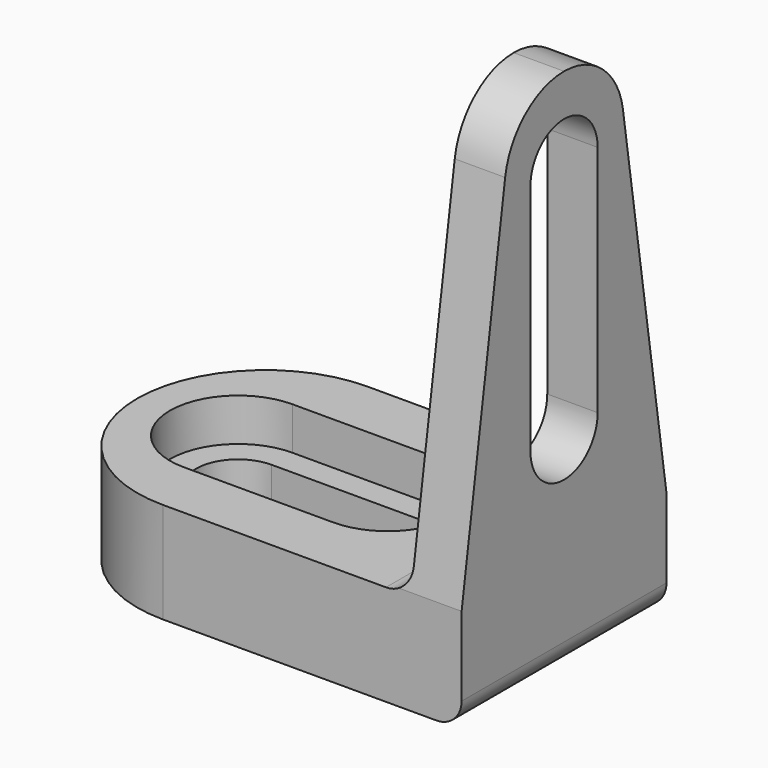
from build123d import *

# Parameters (mm, degrees)
F1_DEPTH    = 15.24
F3_DEPTH    = 3
F5_DEPTH    = 2.54
F6_DEPTH    = 6
F7_C1_SIZE2 = 3.81
F7_C1_SIZE  = 25.1924509954
F7_C2_SIZE2 = 3.81
F7_C2_SIZE  = 25.1924509954
F8_T1_DEPTH = 22.1165158115
F9_R        = 7.61999


# Not quite as in the source:
# - a fillet or chamfer that OpenCascade refuses, or shapes differently, is made with other operations: its cross-section is extruded or revolved along the edge and cut away or added
# - a fillet or chamfer is up to 0.001 mm smaller than in the source, because OpenCascade refuses the exact size


with BuildPart() as f1:
    # F0 (on Front) → F1 (new body)
    with BuildSketch(Plane.XZ):
        with BuildLine():
            ThreePointArc((-3, 4.5), (-3.4393398282, 3.4393398282), (-4.5, 3))
            Line((-4.5, 3), (-25.4, 3))
            Line((-25.4, 3), (-25.4, -3))
            Line((-25.4, -3), (-1.5, -3))
            ThreePointArc((-1.5, -3), (-0.4393398282, -2.5606601718), (0, -1.5))
            Line((0, -1.5), (0, 28.4))
            Line((0, 28.4), (-3, 28.4))
            Line((-3, 28.4), (-3, 4.5))
        make_face()
    extrude(amount=F1_DEPTH)

    # F2 (on face) → F3 (cut, through all)
    with BuildSketch(Plane.YZ):
        with BuildLine():
            ThreePointArc((-5.12, 23.4), (-7.62, 25.9), (-10.12, 23.4))
            Line((-10.12, 23.4), (-10.12, 9.5))
            ThreePointArc((-10.12, 9.5), (-7.62, 7), (-5.12, 9.5))
            Line((-5.12, 9.5), (-5.12, 23.4))
        make_face()
    extrude(amount=-F3_DEPTH, mode=Mode.SUBTRACT)

    # F4 (on face) → F5 (cut)
    with BuildSketch(Plane.XY.offset(3)):
        with BuildLine():
            ThreePointArc((-19.4, -3.57), (-23.45, -7.62), (-19.4, -11.67))
            Line((-19.4, -11.67), (-10.5, -11.67))
            ThreePointArc((-10.5, -11.67), (-6.45, -7.62), (-10.5, -3.57))
            Line((-10.5, -3.57), (-19.4, -3.57))
        make_face()
        with BuildLine():
            Line((-10.5, -10.12), (-19.4, -10.12))
            ThreePointArc((-19.4, -10.12), (-21.9, -7.62), (-19.4, -5.12))
            Line((-19.4, -5.12), (-10.5, -5.12))
            ThreePointArc((-10.5, -5.12), (-8, -7.62), (-10.5, -10.12))
        make_face(mode=Mode.SUBTRACT)
    extrude(amount=-F5_DEPTH, mode=Mode.SUBTRACT)

    # F6 (cut, through all): a face of the model
    f6_faces = [f1.faces().sort_by_distance(p)[0] for p in [
        (-14.95, -7.62, 3),
    ]]
    extrude(f6_faces, amount=-F6_DEPTH, mode=Mode.SUBTRACT)

    # F7: chamfer of 3.81 x 25.1924509954 on 2 edges, made by hand

    # F7_c1
    f7_c1_edges = [f1.edges().sort_by_distance(p)[0] for p in [
        (-1.5, 0, 28.4),
    ]]
    f7_c1_side = f1.faces().sort_by_distance((-1.5, 0, 28.3238))[0]
    chamfer(f7_c1_edges, length=F7_C1_SIZE, length2=F7_C1_SIZE2, reference=f7_c1_side)

    # F7_c2
    f7_c2_edges = [f1.edges().sort_by_distance(p)[0] for p in [
        (-1.5, -15.24, 28.4),
    ]]
    f7_c2_side = f1.faces().sort_by_distance((-1.5, -15.24, 28.3238))[0]
    chamfer(f7_c2_edges, length=F7_C2_SIZE, length2=F7_C2_SIZE2, reference=f7_c2_side)

    # F8: fillet of radius 4.445 on 2 edges, made by hand

    # F8_s2 → F8_t1 (cut)
    with BuildSketch(Plane.YZ.offset(-12.5582579057)):
        with BuildLine():
            ThreePointArc((-12.0017189515, 24.6196846016), (-10.5052742427, 27.3249071244), (-7.6066968377, 28.4))
            Line((-7.6066968377, 28.4), (-11.43, 28.4))
            Line((-11.43, 28.4), (-12.0017189515, 24.6196846016))
        make_face()
        with BuildLine():
            ThreePointArc((-3.2382810485, 24.6196846016), (-4.7347257573, 27.3249071244), (-7.6333031623, 28.4))
            Line((-7.6333031623, 28.4), (-3.81, 28.4))
            Line((-3.81, 28.4), (-3.2382810485, 24.6196846016))
        make_face()
    extrude(amount=F8_T1_DEPTH, mode=Mode.SUBTRACT)

    # F9 (radius 7.62 in the source; OpenCascade refuses exactly that, so slightly less here)
    f9_edges = [f1.edges().sort_by_distance(p)[0] for p in [
        (-25.4, -15.24, 0),
        (-25.4, 0, 0),
    ]]
    fillet(f9_edges, radius=F9_R)


solid = f1.part
